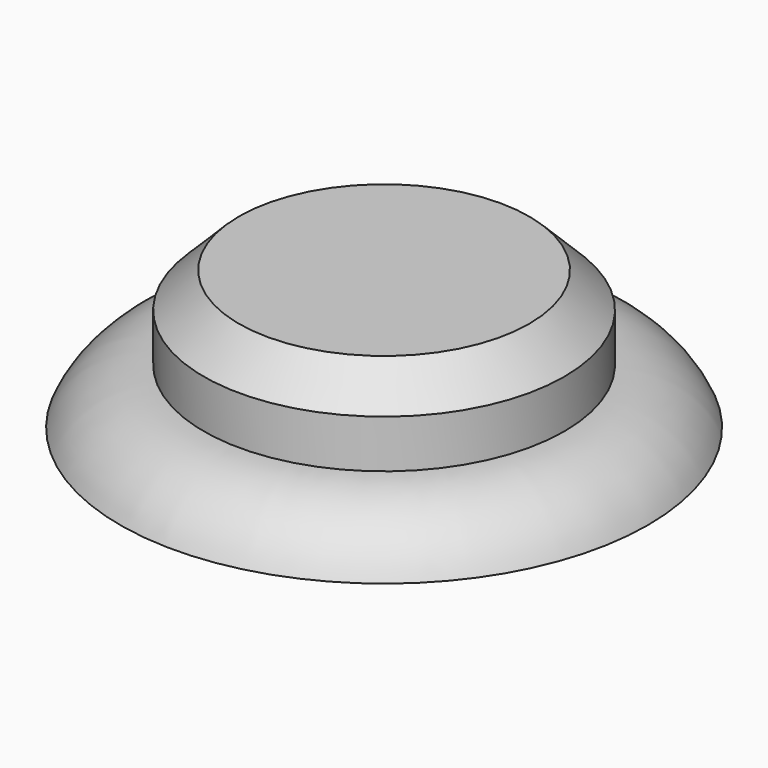
from build123d import *

# Parameters (mm, degrees)
F0_R     = 38.1703800994
F1_DEPTH = 8.0033224076
F3_T     = -5.08
F4_DEPTH = 12.0424441993
F5_SIZE  = 5.08


# Not quite as in the source:
# - a fillet or chamfer that OpenCascade refuses, or shapes differently, is made with other operations: its cross-section is extruded or revolved along the edge and cut away or added


with BuildPart() as f1:
    # F0 (on Top) → F1 (new body)
    with BuildSketch(Plane.XY):
        Circle(F0_R)
    extrude(amount=F1_DEPTH)

    # F2: fillet of radius 13.1324976857 on 1 edges, made by hand

    # F2_s1 → F2_t2 (revolve, cut)
    with BuildSketch(Plane.XZ):
        with BuildLine():
            ThreePointArc((38.1703800994, 0), (33.3302233857, 5.821198641), (26.0809609061, 8.0033224076))
            Line((26.0809609061, 8.0033224076), (38.1703800994, 8.0033224076))
            Line((38.1703800994, 8.0033224076), (38.1703800994, 0))
        make_face()
    revolve(axis=Axis((0, 0, 8.0033224076), (0, 0, 1)), mode=Mode.SUBTRACT)

    # F3
    f3_openings = [f1.faces().sort_by_distance(p)[0] for p in [
        (0, 0, 0),
    ]]
    offset(amount=F3_T, openings=f3_openings)

    # F4 (add): a face of the model
    f4_faces = [f1.faces().sort_by_distance(p)[0] for p in [
        (0, 0, 8.0033224076),
    ]]
    extrude(f4_faces, amount=F4_DEPTH)

    # F5
    f5_edges = [f1.edges().sort_by_distance(p)[0] for p in [
        (-26.080961, 0, 20.045767),
    ]]
    chamfer(f5_edges, length=F5_SIZE)


solid = f1.part
